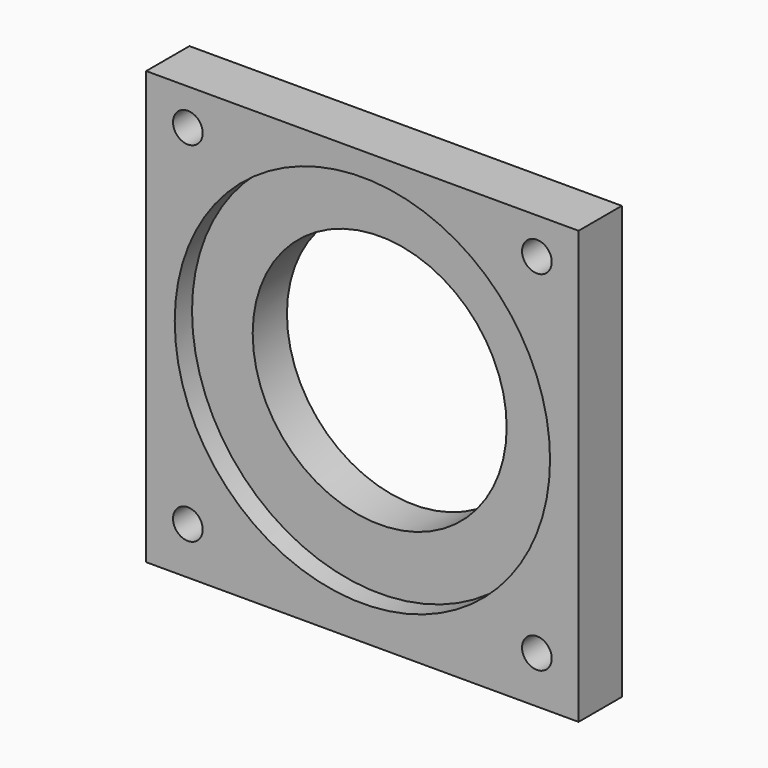
from build123d import *

# Parameters (mm, degrees)
F0_W     = 127
F0_H     = 127
F2_DEPTH = 15.875
F3_R     = 37.2999
F4_DEPTH = 16.002
F5_R     = 55.118
F5_R_2   = 37.2999
F6_DEPTH = 6.35
F7_R     = 54.9275
F7_R_2   = 37.2999
F8_DEPTH = 3.048
F10_D    = 8.73125


# Not quite as in the source:
# - a length typed as a fraction of an inch, garbled in the dataset ("3 / 203.2 mm" for 3/8 in), is restored


with BuildPart() as f2:
    # F0 (on Front) → F2 (new body)
    with BuildSketch(Plane.XZ):
        with Locations((-63.5, 63.5)):
            Rectangle(F0_W, F0_H)
    extrude(amount=F2_DEPTH)

    # F3 (on face) → F4 (cut)
    with BuildSketch(Plane.XZ.offset(15.875)):
        with Locations((-63.5, 65.0875)):
            Circle(F3_R)
    extrude(amount=-F4_DEPTH, mode=Mode.SUBTRACT)

    # F5 (on face) → F6 (cut)
    with BuildSketch(Plane.XZ.offset(15.875)):
        with Locations((-63.5, 65.0875)):
            Circle(F5_R)
        with Locations((-63.5, 65.0875)):
            Circle(F5_R_2, mode=Mode.SUBTRACT)
    extrude(amount=-F6_DEPTH, mode=Mode.SUBTRACT)

    # F7 (on face) → F8 (join)
    with BuildSketch(Plane.XZ):
        with Locations((-63.5, 65.0875)):
            Circle(F7_R)
        with Locations((-63.5, 65.0875)):
            Circle(F7_R_2, mode=Mode.SUBTRACT)
    extrude(amount=-F8_DEPTH)

    # F10 (through all)
    with Locations(Plane.XZ.offset(15.875)):
        with Locations((-114.7572, 116.3447), (-12.2428, 116.3447), (-12.2428, 13.8303), (-114.7572, 13.8303)):
            Hole(F10_D / 2)


solid = f2.part
